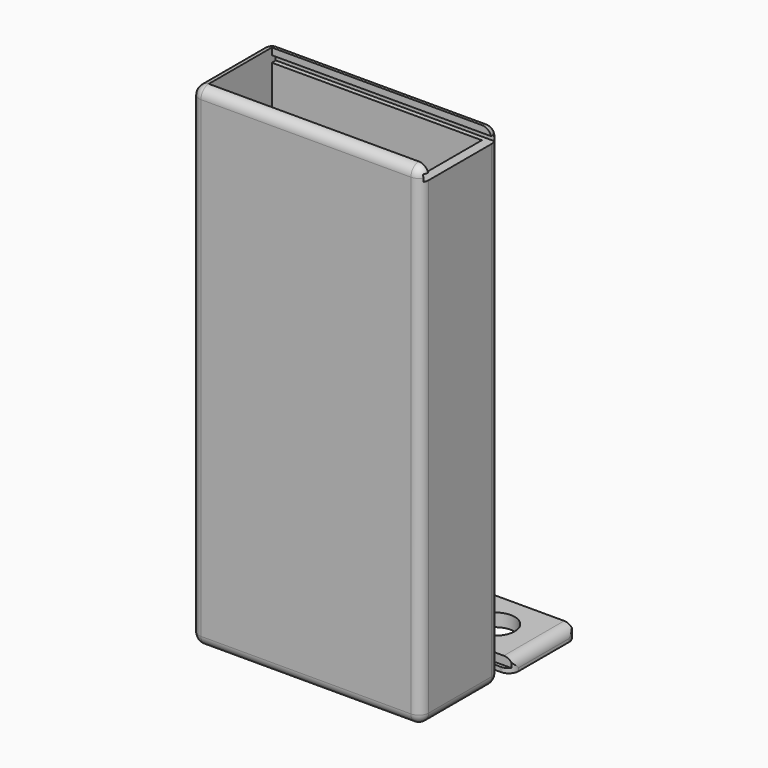
from build123d import *

# Parameters (mm, degrees)
F0_W          = 70
F0_H          = 30
F1_DEPTH      = 150
F2_T          = -3
F3_W          = 24
F3_H          = 2.5384937525
F3_H_2        = 0.4615062475
F4_DEPTH      = 36.4
F4_DEPTH_BACK = 32
F5_R          = 3
F6_R          = 2.9999
F7_W          = 23
F7_H          = 2.5571812009
F7_H_2        = 0.0428187991
F8_DEPTH      = 35
F8_DEPTH_BACK = 31
F9_T1_DEPTH   = 38
F9_T3_DEPTH   = 16.4
F10_R         = 6
F11_DEPTH     = 4.2246429837


# Not quite as in the source:
# - a fillet or chamfer that OpenCascade refuses, or shapes differently, is made with other operations: its cross-section is extruded or revolved along the edge and cut away or added
# - a fillet or chamfer is up to 0.001 mm smaller than in the source, because OpenCascade refuses the exact size


with BuildPart() as f1:
    # F0 (on Top) → F1 (new body)
    with BuildSketch(Plane.XY):
        Rectangle(F0_W, F0_H)
    extrude(amount=F1_DEPTH)

    # F2
    f2_openings = [f1.faces().sort_by_distance(p)[0] for p in [
        (0, 0, 150),
    ]]
    offset(amount=F2_T, openings=f2_openings)

    # F3 (on Right) → F4 (cut, two sides)
    with BuildSketch(Plane.YZ) as f4_sk:
        with Locations((0, 149.2011186481)):
            Rectangle(F3_W, F3_H)
        Polygon((13.5, 147.9318717718), (12, 147.9318717718), (12, 147.4703655243), (-12, 147.4703655243), (-12, 147.9318717718), (-13.5, 147.9318717718), (-13.5, 145.9318717718), (13.5, 145.9318717718), align=None)
        with Locations((0, 147.7011186481)):
            Rectangle(F3_W, F3_H_2)
    extrude(amount=F4_DEPTH, mode=Mode.SUBTRACT)
    extrude(f4_sk.sketch, amount=-F4_DEPTH_BACK, mode=Mode.SUBTRACT)

    # F5
    f5_edges = [f1.edges().sort_by_distance(p)[0] for p in [
        (35, 15, 75),
        (35, -15, 75),
        (35, 0, 0),
        (-35, 0, 0),
        (0, -15, 0),
        (0, 15, 0),
        (-35, 15, 75),
        (-35, -15, 75),
    ]]
    fillet(f5_edges, radius=F5_R)

    # F6 (radius 3 in the source; OpenCascade refuses exactly that, so slightly less here)
    f6_edges = [f1.edges().sort_by_distance(p)[0] for p in [
        (0, -15, 150),
    ]]
    fillet(f6_edges, radius=F6_R)


with BuildPart() as f8:
    # F7 (on Right) → F8 (new body, two sides)
    with BuildSketch(Plane.YZ) as f8_sk:
        with Locations((31.8773090839, 2.9450523832)):
            Rectangle(F7_W, F7_H)
        Polygon((44.4773090839, 1.6664617828), (43.3773090839, 1.6664617828), (43.3773090839, 1.6236429837), (20.3773090839, 1.6236429837), (20.3773090839, 1.6664617828), (19.2773090839, 1.6664617828), (19.2773090839, 0.2664617828), (44.4773090839, 0.2664617828), align=None)
        with Locations((31.8773090839, 1.6450523832)):
            Rectangle(F7_W, F7_H_2)
    extrude(amount=F8_DEPTH)
    extrude(f8_sk.sketch, amount=-F8_DEPTH_BACK)

    # F9: fillet of radius 3 on 3 edges, made by hand

    # F9_s2 → F9_t1 (cut)
    with BuildSketch(Plane.XZ.offset(-50.8773090839)):
        with BuildLine():
            ThreePointArc((35, 1.2236429837), (34.1213203436, 3.3449633272), (32, 4.2236429837))
            Line((32, 4.2236429837), (35, 4.2236429837))
            Line((35, 4.2236429837), (35, 1.2236429837))
        make_face()
    extrude(amount=F9_T1_DEPTH, mode=Mode.SUBTRACT)

    # F9_s4 → F9_t3 (cut)
    with BuildSketch(Plane.XY.offset(-7.2335382172)):
        with BuildLine():
            ThreePointArc((32, 19.2773090839), (34.1213203436, 20.1559887404), (35, 22.2773090839))
            Line((35, 22.2773090839), (35, 19.2773090839))
            Line((35, 19.2773090839), (32, 19.2773090839))
        make_face()
        with BuildLine():
            ThreePointArc((32, 44.4773090839), (34.1213203436, 43.5986294275), (35, 41.4773090839))
            Line((35, 41.4773090839), (35, 44.4773090839))
            Line((35, 44.4773090839), (32, 44.4773090839))
        make_face()
    extrude(amount=F9_T3_DEPTH, mode=Mode.SUBTRACT)

    # F10 (on face) → F11 (cut, through all)
    with BuildSketch(Plane.XY.offset(4.2236429837)):
        with Locations((20.1958809048, 31.8059250712)):
            Circle(F10_R)
    extrude(amount=-F11_DEPTH, mode=Mode.SUBTRACT)


solid = Compound([f1.part, f8.part])
